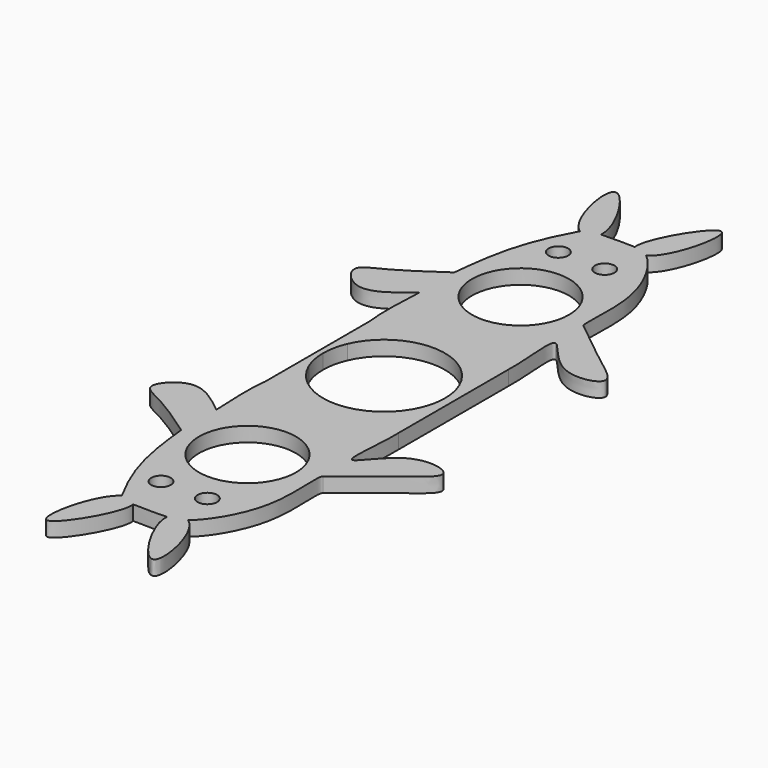
from build123d import *

# Parameters (mm, degrees)
F0_R     = 9.95
F0_R_2   = 2
F1_DEPTH = 3


with BuildPart() as f1:
    # F0 (on Top) → F1 (new body)
    with BuildSketch(Plane.XY):
        with BuildLine():
            ThreePointArc((11.4841992525, 4.9359059482), (12.2434164075, 2.5196735249), (12.5, 0))
            ThreePointArc((12.5, 0), (12.2434164075, -2.5196735249), (11.4841992525, -4.9359059482))
            add(Edge.make_bspline(
                [(14.2224282026, -14.0928809608), (14.0544920655, -9.8907769593), (12.786453361, -7.4166448155), (11.4841992525, -4.9359059482)],
                knots=[0.8325588202, 0.8325588202, 0.8325588202, 0.8325588202, 1, 1, 1, 1], degree=3))
            Line((14.2224282026, -14.0928809608), (14.2224282026, 14.0928809608))
            add(Edge.make_bspline(
                [(14.2224282026, 14.0928809608), (14.0544920655, 9.8907769593), (12.786453361, 7.4166448155), (11.4841992525, 4.9359059482)],
                knots=[0.8325588202, 0.8325588202, 0.8325588202, 0.8325588202, 1, 1, 1, 1], degree=3))
        make_face()
        with BuildLine():
            ThreePointArc((-11.4841992525, 4.9359059482), (0, 12.5), (11.4841992525, 4.9359059482))
            add(Edge.make_bspline(
                [(14.2224282026, 14.0928809608), (14.0544920655, 9.8907769593), (12.786453361, 7.4166448155), (11.4841992525, 4.9359059482)],
                knots=[0.8325588202, 0.8325588202, 0.8325588202, 0.8325588202, 1, 1, 1, 1], degree=3))
            add(Edge.make_bspline(
                [(14.2224282026, 33.4090046103), (17.2490888751, 31.053920445), (22.9972849489, 26.096831604), (31.8177344645, 20.0637888806), (19.9640756328, 17.3628075785), (12.1914727142, 31.6199203566), (14.4096662851, 18.7779589277), (14.2224282026, 14.0928809608)],
                knots=[0, 0, 0, 0, 0.1913410371, 0.3329271624, 0.4817047499, 0.6458725835, 0.8325588202, 0.8325588202, 0.8325588202, 0.8325588202], degree=3))
            add(Edge.make_bspline(
                [(6.7855482785, 58.7356220744), (9.1373873892, 56.8141843385), (15.7434191997, 47.0784545997), (13.3729768574, 33.6002030956), (14.2224282026, 33.4090046103)],
                knots=[0.3534018687, 0.3534018687, 0.3534018687, 0.3534018687, 0.6548758459, 0.9281252581, 0.9281252581, 0.9281252581, 0.9281252581], degree=3))
            add(Edge.make_bspline(
                [(3.4762175574, 59.9388580104), (3.7176838971, 58.2597836406), (5.3504042624, 57.8229914395), (6.7855482785, 58.7356220744)],
                knots=[0.8268984236, 0.8268984236, 0.8268984236, 0.8268984236, 1, 1, 1, 1], degree=3))
            add(Edge.make_bspline(
                [(-3.4762175574, 59.9388580104), (-0.9132762133, 60), (1.6758513881, 60.0610536656), (3.4762175574, 59.9388580104)],
                knots=[0, 0, 0, 0, 0.2064654422, 0.2064654422, 0.2064654422, 0.2064654422], degree=3))
            add(Edge.make_bspline(
                [(-3.4762175574, 59.9388580104), (-3.7176838971, 58.2597836406), (-5.3504042624, 57.8229914395), (-6.7855482785, 58.7356220744)],
                knots=[0.8268984236, 0.8268984236, 0.8268984236, 0.8268984236, 1, 1, 1, 1], degree=3))
            add(Edge.make_bspline(
                [(-6.7855482785, 58.7356220744), (-8.5881051608, 55.5003900744), (-12.1208026299, 47.809859872), (-13.1336634583, 39.352034704), (-13.5873220861, 35)],
                knots=[0, 0, 0, 0, 0.4891254011, 1, 1, 1, 1], degree=3))
            add(Edge.make_bspline(
                [(-13.5873220861, 35), (-16.9512808708, 32.6719958826), (-22.4422707428, 28.8719947978), (-28.7100144619, 26.5342926433), (-22.0598012934, 19.1597220145), (-16.6324705303, 23.5247038367), (-13.5873220861, 25.9737931192)],
                knots=[0, 0, 0, 0, 0.3038929296, 0.4960444243, 0.7172423049, 1, 1, 1, 1], degree=3))
            add(Edge.make_bspline(
                [(-13.5873220861, 25.9737931192), (-13.7484282726, 21.5353356165), (-14.1021202558, 17.0585195355), (-13.5873220861, 13.4542575106)],
                knots=[0, 0, 0, 0, 0.544318651, 0.544318651, 0.544318651, 0.544318651], degree=3))
            add(Edge.make_bspline(
                [(-13.5873220861, 13.4542575106), (-13.1563540785, 10.436916512), (-12.116717364, 8.0310923479), (-11.4841992525, 4.9359059482)],
                knots=[0.544318651, 0.544318651, 0.544318651, 0.544318651, 1, 1, 1, 1], degree=3))
        make_face()
        with Locations((0, 35)):
            Circle(F0_R, mode=Mode.SUBTRACT)
        with Locations((-4.9894000404, 50.9333796799)):
            Circle(F0_R_2, mode=Mode.SUBTRACT)
        with Locations((4.5164329931, 50.9333796799)):
            Circle(F0_R_2, mode=Mode.SUBTRACT)
        with BuildLine():
            add(Edge.make_bspline(
                [(14.2224282026, -14.0928809608), (14.0544920655, -9.8907769593), (12.786453361, -7.4166448155), (11.4841992525, -4.9359059482)],
                knots=[0.8325588202, 0.8325588202, 0.8325588202, 0.8325588202, 1, 1, 1, 1], degree=3))
            ThreePointArc((11.4841992525, -4.9359059482), (0, -12.5), (-11.4841992525, -4.9359059482))
            add(Edge.make_bspline(
                [(-13.5873220861, -13.4542575106), (-13.1563540785, -10.436916512), (-12.116717364, -8.0310923479), (-11.4841992525, -4.9359059482)],
                knots=[0.544318651, 0.544318651, 0.544318651, 0.544318651, 1, 1, 1, 1], degree=3))
            add(Edge.make_bspline(
                [(-13.5873220861, -25.9737931192), (-13.7484282726, -21.5353356165), (-14.1021202558, -17.0585195355), (-13.5873220861, -13.4542575106)],
                knots=[0, 0, 0, 0, 0.544318651, 0.544318651, 0.544318651, 0.544318651], degree=3))
            add(Edge.make_bspline(
                [(-13.5873220861, -35), (-16.9512808708, -32.6719958826), (-22.4422707428, -28.8719947978), (-28.7100144619, -26.5342926433), (-22.0598012934, -19.1597220145), (-16.6324705303, -23.5247038367), (-13.5873220861, -25.9737931192)],
                knots=[0, 0, 0, 0, 0.3038929296, 0.4960444243, 0.7172423049, 1, 1, 1, 1], degree=3))
            add(Edge.make_bspline(
                [(-6.7855482785, -58.7356220744), (-8.5881051608, -55.5003900744), (-12.1208026299, -47.809859872), (-13.1336634583, -39.352034704), (-13.5873220861, -35)],
                knots=[0, 0, 0, 0, 0.4891254011, 1, 1, 1, 1], degree=3))
            add(Edge.make_bspline(
                [(-3.4762175574, -59.9388580104), (-3.7176838971, -58.2597836406), (-5.3504042624, -57.8229914395), (-6.7855482785, -58.7356220744)],
                knots=[0.8268984236, 0.8268984236, 0.8268984236, 0.8268984236, 1, 1, 1, 1], degree=3))
            add(Edge.make_bspline(
                [(-3.4762175574, -59.9388580104), (-0.9132762133, -60), (1.6758513881, -60.0610536656), (3.4762175574, -59.9388580104)],
                knots=[0, 0, 0, 0, 0.2064654422, 0.2064654422, 0.2064654422, 0.2064654422], degree=3))
            add(Edge.make_bspline(
                [(3.4762175574, -59.9388580104), (3.7176838971, -58.2597836406), (5.3504042624, -57.8229914395), (6.7855482785, -58.7356220744)],
                knots=[0.8268984236, 0.8268984236, 0.8268984236, 0.8268984236, 1, 1, 1, 1], degree=3))
            add(Edge.make_bspline(
                [(6.7855482785, -58.7356220744), (9.1373873892, -56.8141843385), (15.7434191997, -47.0784545997), (13.3729768574, -33.6002030956), (14.2224282026, -33.4090046103)],
                knots=[0.3534018687, 0.3534018687, 0.3534018687, 0.3534018687, 0.6548758459, 0.9281252581, 0.9281252581, 0.9281252581, 0.9281252581], degree=3))
            add(Edge.make_bspline(
                [(14.2224282026, -33.4090046103), (17.2490888751, -31.053920445), (22.9972849489, -26.096831604), (31.8177344645, -20.0637888806), (19.9640756328, -17.3628075785), (12.1914727142, -31.6199203566), (14.4096662851, -18.7779589277), (14.2224282026, -14.0928809608)],
                knots=[0, 0, 0, 0, 0.1913410371, 0.3329271624, 0.4817047499, 0.6458725835, 0.8325588202, 0.8325588202, 0.8325588202, 0.8325588202], degree=3))
        make_face()
        with Locations((-4.9894000404, -50.9333796799)):
            Circle(F0_R_2, mode=Mode.SUBTRACT)
        with Locations((0, -35)):
            Circle(F0_R, mode=Mode.SUBTRACT)
        with Locations((4.5164329931, -50.9333796799)):
            Circle(F0_R_2, mode=Mode.SUBTRACT)
        with BuildLine():
            ThreePointArc((-12.5, 0), (-12.2434164075, 2.5196735249), (-11.4841992525, 4.9359059482))
            add(Edge.make_bspline(
                [(-13.5873220861, 13.4542575106), (-13.1563540785, 10.436916512), (-12.116717364, 8.0310923479), (-11.4841992525, 4.9359059482)],
                knots=[0.544318651, 0.544318651, 0.544318651, 0.544318651, 1, 1, 1, 1], degree=3))
            Line((-13.5873220861, 13.4542575106), (-13.5873220861, -13.4542575106))
            add(Edge.make_bspline(
                [(-13.5873220861, -13.4542575106), (-13.1563540785, -10.436916512), (-12.116717364, -8.0310923479), (-11.4841992525, -4.9359059482)],
                knots=[0.544318651, 0.544318651, 0.544318651, 0.544318651, 1, 1, 1, 1], degree=3))
            ThreePointArc((-11.4841992525, -4.9359059482), (-12.2434164075, -2.5196735249), (-12.5, 0))
        make_face()
        with BuildLine():
            add(Edge.make_bspline(
                [(3.4762175574, 59.9388580104), (4.75749431, 59.8518943387), (5.6392774199, 59.6721181439), (6.7855482785, 58.7356220744)],
                knots=[0.2064654422, 0.2064654422, 0.2064654422, 0.2064654422, 0.3534018687, 0.3534018687, 0.3534018687, 0.3534018687], degree=3))
            add(Edge.make_bspline(
                [(6.7855482785, 58.7356220744), (9.5293676869, 60.4804599584), (12.4284956458, 70.0561754003), (10.4054106349, 75.4105917089), (2.9847830091, 63.356125839), (3.4762175574, 59.9388580104)],
                knots=[0, 0, 0, 0, 0.3309489915, 0.4746004798, 0.8268984236, 0.8268984236, 0.8268984236, 0.8268984236], degree=3))
        make_face()
        with BuildLine():
            add(Edge.make_bspline(
                [(3.4762175574, 59.9388580104), (3.7176838971, 58.2597836406), (5.3504042624, 57.8229914395), (6.7855482785, 58.7356220744)],
                knots=[0.8268984236, 0.8268984236, 0.8268984236, 0.8268984236, 1, 1, 1, 1], degree=3))
            add(Edge.make_bspline(
                [(3.4762175574, 59.9388580104), (4.75749431, 59.8518943387), (5.6392774199, 59.6721181439), (6.7855482785, 58.7356220744)],
                knots=[0.2064654422, 0.2064654422, 0.2064654422, 0.2064654422, 0.3534018687, 0.3534018687, 0.3534018687, 0.3534018687], degree=3))
        make_face()
        with BuildLine():
            add(Edge.make_bspline(
                [(6.7855482785, -58.7356220744), (9.5293676869, -60.4804599584), (12.4284956458, -70.0561754003), (10.4054106349, -75.4105917089), (2.9847830091, -63.356125839), (3.4762175574, -59.9388580104)],
                knots=[0, 0, 0, 0, 0.3309489915, 0.4746004798, 0.8268984236, 0.8268984236, 0.8268984236, 0.8268984236], degree=3))
            add(Edge.make_bspline(
                [(3.4762175574, -59.9388580104), (4.75749431, -59.8518943387), (5.6392774199, -59.6721181439), (6.7855482785, -58.7356220744)],
                knots=[0.2064654422, 0.2064654422, 0.2064654422, 0.2064654422, 0.3534018687, 0.3534018687, 0.3534018687, 0.3534018687], degree=3))
        make_face()
        with BuildLine():
            add(Edge.make_bspline(
                [(3.4762175574, -59.9388580104), (4.75749431, -59.8518943387), (5.6392774199, -59.6721181439), (6.7855482785, -58.7356220744)],
                knots=[0.2064654422, 0.2064654422, 0.2064654422, 0.2064654422, 0.3534018687, 0.3534018687, 0.3534018687, 0.3534018687], degree=3))
            add(Edge.make_bspline(
                [(3.4762175574, -59.9388580104), (3.7176838971, -58.2597836406), (5.3504042624, -57.8229914395), (6.7855482785, -58.7356220744)],
                knots=[0.8268984236, 0.8268984236, 0.8268984236, 0.8268984236, 1, 1, 1, 1], degree=3))
        make_face()
        with BuildLine():
            add(Edge.make_bspline(
                [(-6.7855482785, 58.7356220744), (-9.5293676869, 60.4804599584), (-12.4284956458, 70.0561754003), (-10.4054106349, 75.4105917089), (-2.9847830091, 63.356125839), (-3.4762175574, 59.9388580104)],
                knots=[0, 0, 0, 0, 0.3309489915, 0.4746004798, 0.8268984236, 0.8268984236, 0.8268984236, 0.8268984236], degree=3))
            add(Edge.make_bspline(
                [(-3.4762175574, 59.9388580104), (-3.7176838971, 58.2597836406), (-5.3504042624, 57.8229914395), (-6.7855482785, 58.7356220744)],
                knots=[0.8268984236, 0.8268984236, 0.8268984236, 0.8268984236, 1, 1, 1, 1], degree=3))
        make_face()
        with BuildLine():
            add(Edge.make_bspline(
                [(-6.7855482785, -58.7356220744), (-9.5293676869, -60.4804599584), (-12.4284956458, -70.0561754003), (-10.4054106349, -75.4105917089), (-2.9847830091, -63.356125839), (-3.4762175574, -59.9388580104)],
                knots=[0, 0, 0, 0, 0.3309489915, 0.4746004798, 0.8268984236, 0.8268984236, 0.8268984236, 0.8268984236], degree=3))
            add(Edge.make_bspline(
                [(-3.4762175574, -59.9388580104), (-3.7176838971, -58.2597836406), (-5.3504042624, -57.8229914395), (-6.7855482785, -58.7356220744)],
                knots=[0.8268984236, 0.8268984236, 0.8268984236, 0.8268984236, 1, 1, 1, 1], degree=3))
        make_face()
    extrude(amount=F1_DEPTH)


solid = f1.part
